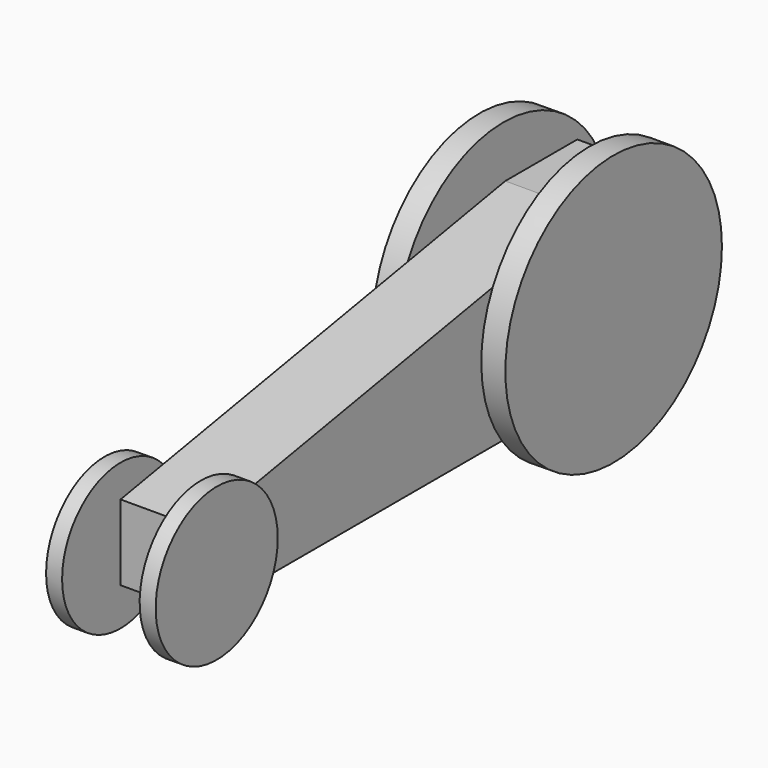
from build123d import *

# Parameters (mm, degrees)
F0_R         = 42.8944136966
F1_DEPTH     = 7.62
F2_W         = 53.9315019637
F2_H         = 50.8
F3_DEPTH     = 25.4
F4_DEPTH     = 127
F5_R         = 42.3296228718
F6_DEPTH     = 7.62
F7_R         = 23.1378072787
F8_DEPTH     = 5.08
F9_R         = 24.1805765137
F10_DEPTH    = 5.08
F11_T1_DEPTH = 25.4


# Not quite as in the source:
# - a fillet or chamfer that OpenCascade refuses, or shapes differently, is made with other operations: its cross-section is extruded or revolved along the edge and cut away or added


with BuildPart() as f1:
    # F0 (on Right) → F1 (new body)
    with BuildSketch(Plane.YZ):
        Circle(F0_R)
    extrude(amount=F1_DEPTH)

    # F2 (on face) → F3 (join)
    with BuildSketch(Plane(origin=(0, 0, 0), x_dir=(0, -1, 0), z_dir=(-1, 0, 0))):
        with Locations((0.0807167962, 0.2214573324)):
            Rectangle(F2_W, F2_H)
    extrude(amount=F3_DEPTH)

    # F4 (add): a face of the model
    f4_faces = [f1.faces().sort_by_distance(p)[0] for p in [
        (-12.7, -27.0464677781, 0.2214573324),
    ]]
    extrude(f4_faces, amount=F4_DEPTH)

    # F5 (on face) → F6 (join)
    with BuildSketch(Plane(origin=(-25.4, 0, 0), x_dir=(0, -1, 0), z_dir=(-1, 0, 0))):
        with Locations((2.3584635928, 0)):
            Circle(F5_R)
    extrude(amount=F6_DEPTH)

    # F7 (on face) → F8 (join)
    with BuildSketch(Plane(origin=(-25.4, 0, 0), x_dir=(0, -1, 0), z_dir=(-1, 0, 0))):
        with Locations((154.0464677781, -14.1031453386)):
            Circle(F7_R)
    extrude(amount=F8_DEPTH)

    # F9 (on face) → F10 (join)
    with BuildSketch(Plane.YZ):
        with Locations((-154.0464677781, -11.9213024154)):
            Circle(F9_R)
    extrude(amount=F10_DEPTH)

    # F11: chamfer of 152.4 x 26.87223186 on 1 edges, made by hand

    # F11_s2 → F11_t1 (cut)
    with BuildSketch(Plane.YZ.offset(-25.4)):
        Polygon((-1.6464677781, 25.6214573324), (-154.0464677781, -1.2507745276), (-154.0464677781, 25.6214573324), align=None)
    extrude(amount=F11_T1_DEPTH, mode=Mode.SUBTRACT)


solid = f1.part
